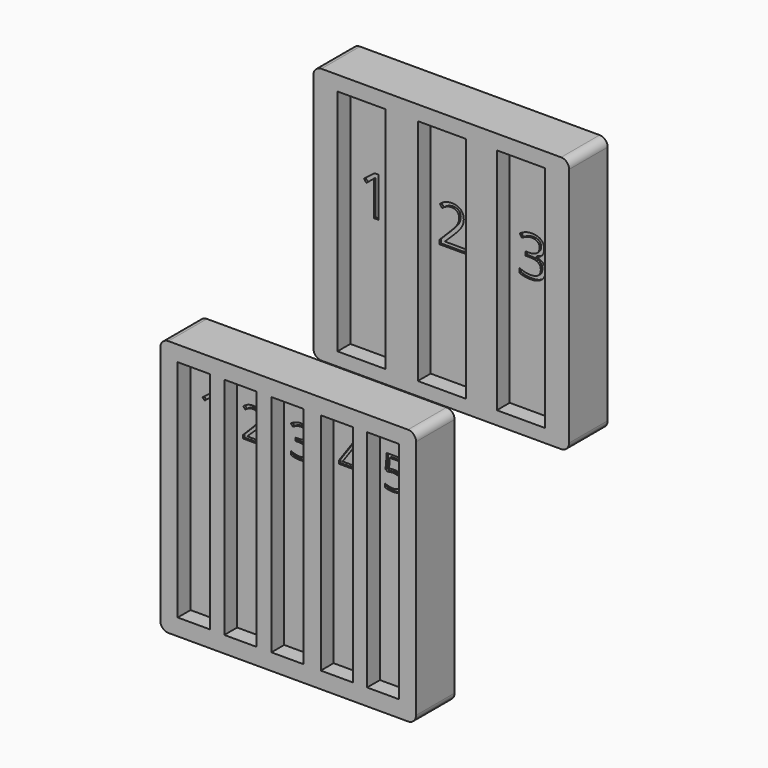
from build123d import *

# Parameters (mm, degrees)
F0_W          = 63.7
F0_H          = 64
F1_DEPTH      = 12
F2_W          = 8
F2_H          = 56
F3_DEPTH      = 4
F4_TEXT_SIZE  = 11.1111111111
F5_DEPTH      = 0.5
F6_W          = 63.7
F6_H          = 64
F7_DEPTH      = 12
F8_W          = 12
F8_H          = 57
F9_DEPTH      = 4
F10_TEXT_SIZE = 13.8888888889
F11_DEPTH     = 0.5
F12_R         = 2
F15_R         = 2


# Not quite as in the source:
# - Text() gives the source's letters only with a copy of the font that has no kerning and outlines rounded to 1/6400 em; it was checked with that copy


with BuildPart() as f1:
    # F0 (on Front) → F1 (new body)
    with BuildSketch(Plane.XZ):
        with Locations((-3.3642866403, 1.4523437072)):
            Rectangle(F0_W, F0_H)
    extrude(amount=F1_DEPTH)

    # F2 (on face) → F3 (cut)
    with BuildSketch(Plane.XZ.offset(12)):
        with Locations((-26.8928594887, 1.594719193)):
            Rectangle(F2_W, F2_H)
        with Locations((-15.278571941, 1.5428709537)):
            Rectangle(F2_W, F2_H)
        with Locations((-3.5499989616, 1.5428709537)):
            Rectangle(F2_W, F2_H)
        with Locations((8.7499981439, 1.5428709537)):
            Rectangle(F2_W, F2_H)
        with Locations((20.2928607315, 1.5895969719)):
            Rectangle(F2_W, F2_H)
    extrude(amount=-F3_DEPTH, mode=Mode.SUBTRACT)

    # F4 (on face) → F5 (cut)
    with BuildSketch(Plane.XZ.offset(8)):
        with Locations((-28.8958736829, 14.9612163462)):
            Text('1', F4_TEXT_SIZE, font='Open Sans', text_align=(TextAlign.LEFT, TextAlign.BOTTOM))
        with Locations((-18.3880866883, 15.4684507965)):
            Text('2', F4_TEXT_SIZE, font='Open Sans', text_align=(TextAlign.LEFT, TextAlign.BOTTOM))
        with Locations((-6.421875, 15.4684507965)):
            Text('3', F4_TEXT_SIZE, font='Open Sans', text_align=(TextAlign.LEFT, TextAlign.BOTTOM))
        with Locations((5.8542882737, 15.8708592951)):
            Text('4', F4_TEXT_SIZE, font='Open Sans', text_align=(TextAlign.LEFT, TextAlign.BOTTOM))
        with Locations((16.7789870777, 16.0218453109)):
            Text('5', F4_TEXT_SIZE, font='Open Sans', text_align=(TextAlign.LEFT, TextAlign.BOTTOM))
    extrude(amount=-F5_DEPTH, mode=Mode.SUBTRACT)


with BuildPart() as f7:
    # F6 (on Front) → F7 (new body)
    with BuildSketch(Plane.XZ):
        with Locations((-3.7279066384, 11.6875871464)):
            Rectangle(F6_W, F6_H)
    extrude(amount=F7_DEPTH)

    # F8 (on face) → F9 (cut)
    with BuildSketch(Plane.XZ.offset(12)):
        with Locations((-23.5779066384, 11.5155177418)):
            Rectangle(F8_W, F8_H)
        with Locations((-3.5779062063, 11.5155177418)):
            Rectangle(F8_W, F8_H)
        with Locations((16.1220933616, 11.5155177418)):
            Rectangle(F8_W, F8_H)
    extrude(amount=-F9_DEPTH, mode=Mode.SUBTRACT)

    # F10 (on face) → F11 (cut)
    with BuildSketch(Plane.XZ.offset(8)):
        with Locations((-27.4568052245, 12.5000027567)):
            Text('1', F10_TEXT_SIZE, font='Open Sans', text_align=(TextAlign.LEFT, TextAlign.BOTTOM))
        with Locations((-8.0967881944, 12.0913628815)):
            Text('2', F10_TEXT_SIZE, font='Open Sans', text_align=(TextAlign.LEFT, TextAlign.BOTTOM))
        with Locations((11.9004505929, 11.9228398055)):
            Text('3', F10_TEXT_SIZE, font='Open Sans', text_align=(TextAlign.LEFT, TextAlign.BOTTOM))
    extrude(amount=-F11_DEPTH, mode=Mode.SUBTRACT)

    # F12
    f12_edges = [f7.edges().sort_by_distance(p)[0] for p in [
        (-35.577907, -6, -20.312413),
        (28.122093, -6, -20.312413),
        (28.122093, -6, 43.687587),
        (-35.577907, -6, 43.687587),
    ]]
    fillet(f12_edges, radius=F12_R)


with BuildPart() as f7_1:
    # F13: moved
    add(f7.part.moved(Location((38.5, 0, 40.6))))


with BuildPart() as f1_1:
    # F14: moved
    add(f1.part.moved(Location((0, 0, -21.3))))

    # F15
    f15_edges = [f1_1.edges().sort_by_distance(p)[0] for p in [
        (-35.214287, -6, -51.847656),
        (28.485713, -6, -51.847656),
        (-35.214287, -6, 12.152344),
        (28.485713, -6, 12.152344),
    ]]
    fillet(f15_edges, radius=F15_R)


solid = Compound([f7_1.part, f1_1.part])
